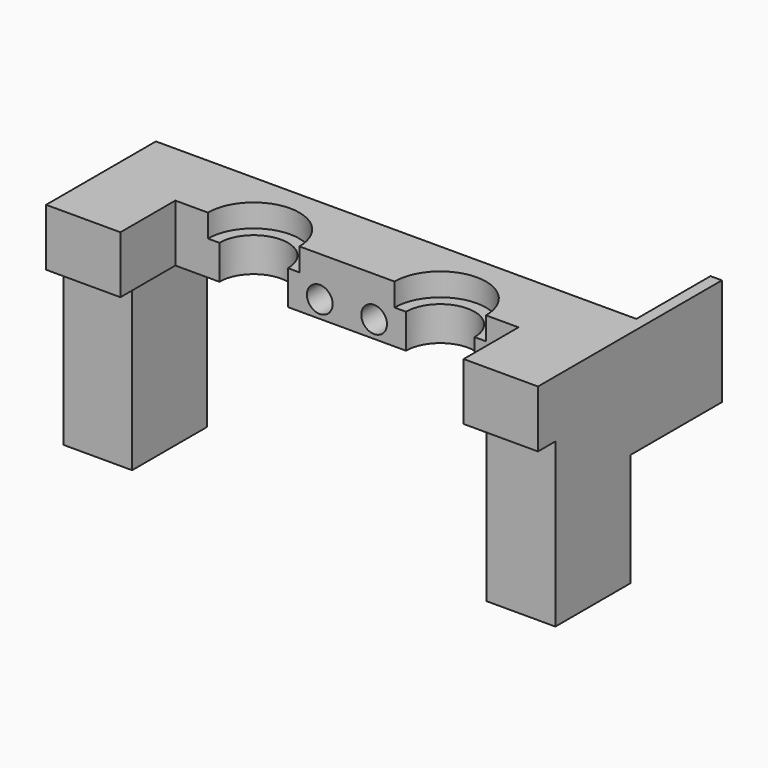
from build123d import *

# Parameters (mm, degrees)
F0_W          = 12
F0_H          = 16.5
F0_R          = 1.6
F1_DEPTH      = 17.5
F5_W          = 12
F5_H          = 16.5
F6_DEPTH      = 3
F2_W          = 12
F2_H          = 16.4
F7_DEPTH      = 35.5
F7_DEPTH_BACK = 3
F11_W         = 50
F11_H         = 5.5
F12_DEPTH     = 90
F14_DEPTH     = 10
F15_R         = 1.5
F16_DEPTH     = 7
F17_R         = 8
F18_DEPTH     = 15
F22_R         = 8
F22_R_2       = 6
F23_DEPTH     = 6
F25_DEPTH     = 25
F26_R         = 2.25
F27_DEPTH     = 25
F28_R         = 2.25
F29_DEPTH     = 3
F30_W         = 20
F30_H         = 18.7556861639
F31_DEPTH     = 2


# Not quite as in the source:
# - a feature of the source that left no trace in its solid (it failed there, or was rolled back) is left out


with BuildPart() as f1:
    # F0 (on Top) → F1 (new body)
    with BuildSketch(Plane.XY):
        Polygon((-43, -44.5), (43, -44.5), (43, -3), (31, -3), (31, -11.5), (-31, -11.5), (-31, -3), (-43, -3), align=None)
        with Locations((37, 5.25)):
            Rectangle(F0_W, F0_H)
        with Locations((37, 5.25)):
            Circle(F0_R, mode=Mode.SUBTRACT)
        with Locations((-37, 5.25)):
            Rectangle(F0_W, F0_H)
        with Locations((-37, 5.25)):
            Circle(F0_R, mode=Mode.SUBTRACT)
        Polygon((31, 13.5), (43, 13.5), (43, 44.5), (-43, 44.5), (-43, 13.5), (-31, 13.5), (-31, 25.5), (31, 25.5), align=None)
    extrude(amount=F1_DEPTH)

    # F5 (on face) → F6 (cut)
    with BuildSketch(Plane.XY.offset(17.5)):
        with Locations((-37, 5.25)):
            Rectangle(F5_W, F5_H)
        with Locations((37, 5.25)):
            Rectangle(F5_W, F5_H)
    extrude(amount=-F6_DEPTH, mode=Mode.SUBTRACT)

    # F11 (on face) → F12 (cut)
    with BuildSketch(Plane(origin=(-43, 0, 0), x_dir=(0, -1, 0), z_dir=(-1, 0, 0))):
        with Locations((0, 2.75)):
            Rectangle(F11_W, F11_H)
    extrude(amount=-F12_DEPTH, mode=Mode.SUBTRACT)


with BuildPart() as f7:
    # F2 (on face) → F7 (new body, two sides)
    with BuildSketch(Plane.XY.offset(17.5)) as f7_sk:
        with Locations((37, 5.25)):
            Rectangle(F2_W, F2_H)
    extrude(amount=F7_DEPTH)
    extrude(f7_sk.sketch, amount=-F7_DEPTH_BACK)



with BuildPart() as f7b:
    # F2 (on face) → F7, piece 2 (new body, two sides)
    with BuildSketch(Plane.XY.offset(17.5)) as f7_2_sk:
        with Locations((-37, 5.25)):
            Rectangle(F2_W, F2_H)
    extrude(amount=F7_DEPTH)
    extrude(f7_2_sk.sketch, amount=-F7_DEPTH_BACK)


with BuildPart() as f7_1:
    add(f7.part)

    add(f7b.part)  # F14 merges F7b
    # F13 (on face) → F14 (join)
    with BuildSketch(Plane.XY.offset(53)):
        Polygon((43, -6.75), (43, 13.5), (43, 17.25), (-43, 17.25), (-43, -6.75), align=None)
    extrude(amount=-F14_DEPTH)

    # F15 (on face) → F16 (cut)
    with BuildSketch(Plane(origin=(0, 0, 14.5), x_dir=(1, 0, 0), z_dir=(0, 0, -1))):
        with Locations((-37, -5.25)):
            Circle(F15_R)
        with Locations((37, -5.25)):
            Circle(F15_R)
    extrude(amount=-F16_DEPTH, mode=Mode.SUBTRACT)

    # F17 (on face) → F18 (cut)
    with BuildSketch(Plane.XY.offset(53)):
        with Locations((16.3168814033, 5.25)):
            Circle(F17_R)
        with Locations((-16.3168814033, 5.25)):
            Circle(F17_R)
    extrude(amount=-F18_DEPTH, mode=Mode.SUBTRACT)

    # F22 (on offset) → F23 (join)
    with BuildSketch(Plane.XY.offset(49)):
        with Locations((-16.3168814033, 5.25)):
            Circle(F22_R)
        with Locations((-16.3168814033, 5.25)):
            Circle(F22_R_2, mode=Mode.SUBTRACT)
        with Locations((16.3168814033, 5.25)):
            Circle(F22_R)
        with Locations((16.3168814033, 5.25)):
            Circle(F22_R_2, mode=Mode.SUBTRACT)
    extrude(amount=-F23_DEPTH)

    # F24 (on face) → F25 (cut)
    with BuildSketch(Plane.XY.offset(53)):
        with BuildLine():
            Line((-30, 5.25), (-30, -6.75))
            Line((-30, -6.75), (30, -6.75))
            Line((30, -6.75), (30, 5.25))
            Line((30, 5.25), (-10.3168814033, 5.25))
            ThreePointArc((-10.3168814033, 5.25), (-16.3168814033, -0.75), (-22.3168814033, 5.25))
            Line((-22.3168814033, 5.25), (-30, 5.25))
        make_face()
        with BuildLine():
            ThreePointArc((-10.3168814033, 5.25), (-16.3168814033, 11.25), (-22.3168814033, 5.25))
            Line((-22.3168814033, 5.25), (-10.3168814033, 5.25))
        make_face()
        with BuildLine():
            Line((-10.3168814033, 5.25), (-22.3168814033, 5.25))
            ThreePointArc((-22.3168814033, 5.25), (-16.3168814033, -0.75), (-10.3168814033, 5.25))
        make_face()
    extrude(amount=-F25_DEPTH, mode=Mode.SUBTRACT)

    # F26 (on face) → F27 (cut)
    with BuildSketch(Plane.XZ.offset(-5.25)):
        with Locations((-4.75, 46)):
            Circle(F26_R)
        with Locations((4.75, 46)):
            Circle(F26_R)
    extrude(amount=-F27_DEPTH, mode=Mode.SUBTRACT)

    # F28 (on face) → F29 (cut)
    with BuildSketch(Plane(origin=(0, 17.25, 0), x_dir=(-1, 0, 0), z_dir=(0, 1, 0))):
        Polygon((8.5, 43.8349364905), (8.5, 48.1650635095), (4.75, 50.3301270189), (1, 48.1650635095), (1, 43.8349364905), (4.75, 41.6698729811), align=None)
        with Locations((4.75, 46)):
            Circle(F28_R, mode=Mode.SUBTRACT)
        Polygon((-1, 43.8349364905), (-1, 48.1650635095), (-4.75, 50.3301270189), (-8.5, 48.1650635095), (-8.5, 43.8349364905), (-4.75, 41.6698729811), align=None)
        with Locations((-4.75, 46)):
            Circle(F28_R, mode=Mode.SUBTRACT)
    extrude(amount=-F29_DEPTH, mode=Mode.SUBTRACT)

    # F30 (on face) → F31 (join)
    with BuildSketch(Plane.YZ.offset(43)):
        with Locations((23.45, 43.622156918)):
            Rectangle(F30_W, F30_H)
    extrude(amount=-F31_DEPTH)


solid = f7_1.part
